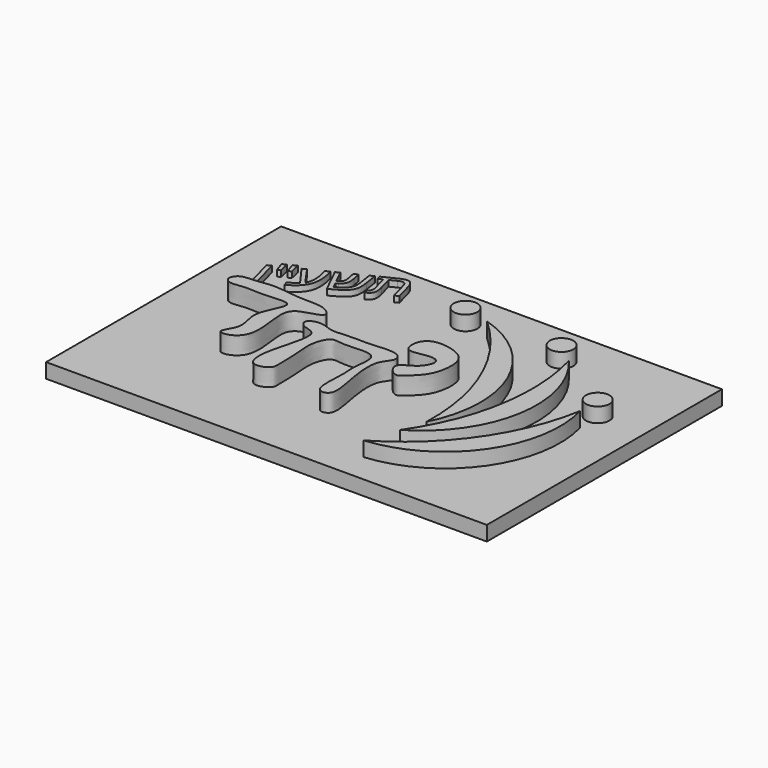
from build123d import *

# Parameters (mm, degrees)
F0_W         = 75
F0_H         = 50
F1_DEPTH     = 2.5
F2_R         = 2
F3_DEPTH     = 2.5
F5_DEPTH     = 3
F6_TEXT_SIZE = 8.2016766118
F7_DEPTH     = 1
F9_W         = 11.5771840792
F9_H         = 10.4032866075
F10_DEPTH    = 0.5


# Not quite as in the source:
# - Text() gives the source's letters only with a copy of the font that has no kerning and outlines rounded to 1/6400 em; it was checked with that copy


with BuildPart() as f1:
    # F0 (on Top) → F1 (new body)
    with BuildSketch(Plane.XY):
        Rectangle(F0_W, F0_H)
    extrude(amount=F1_DEPTH)

    # F2 (on face) → F3 (join)
    with BuildSketch(Plane.XY.offset(2.5)):
        with BuildLine():
            ThreePointArc((29.7072930905, 4.5745613287), (23.8276710869, -9.620101854), (12.5, -20))
            ThreePointArc((12.5, -20), (26.8332996169, -11.7246656078), (29.7072930905, 4.5745613287))
        make_face()
        with BuildLine():
            ThreePointArc((19.5, 14.9611591388), (20.2390516093, -0.3852482744), (14.4231878129, -14.6061535226))
            ThreePointArc((14.4231878129, -14.6061535226), (23.855326069, -1.0061753928), (19.5, 14.9611591388))
        make_face()
        with BuildLine():
            ThreePointArc((3.9204793744, 17), (12.8657059665, 4.5083492287), (15.6936347485, -10.5933472514))
            ThreePointArc((15.6936347485, -10.5933472514), (16.2405516301, 5.9482826301), (3.9204793744, 17))
        make_face()
        with Locations((29.4776950032, 8.6062820628)):
            Circle(F2_R)
        with Locations((15.9142967314, 17.8679712117)):
            Circle(F2_R)
        with Locations((-0.7517675404, 18.2841885835)):
            Circle(F2_R)
    extrude(amount=F3_DEPTH)

    # F4 (on face) → F5 (join)
    with BuildSketch(Plane.XY.offset(2.5)):
        with BuildLine():
            add(Edge.make_bspline(
                [(3.0326086562, -1.3369563967), (2.9350119626, -2.0403621451), (4.5917425614, -3.9939270927), (6.1221765899, -2.3629044841), (8.5639301497, -0.2651330915), (9.1837782901, 4.6769157571), (7.1382724113, 7.1335732235), (0.9439931643, 8.0903867753), (0.6074509574, 2.4736840768), (4.3394964182, 3.7996694306), (7.1189866446, 3.4381517938), (5.7369825883, 0.0853711506), (3.1405351803, -0.5591007677), (3.0326086562, -1.3369563967)],
                knots=[0, 0, 0, 0, 0.0820283677, 0.149981563, 0.2443794271, 0.3552738175, 0.4458566049, 0.5629281656, 0.6566670853, 0.7481320898, 0.8236216622, 0.9092895847, 1, 1, 1, 1], degree=3))
        make_face()
        with BuildLine():
            add(Edge.make_bspline(
                [(-8.1195654348, 1.4021738898), (-7.3091460708, 1.4638883512), (-5.5152173406, 1.4979414066), (-3.8993839761, 1.3561788354), (1.3062373781, 2.0276326248), (2.1890052278, -0.1990991053), (-0.1899071058, -2.0595975618), (0.8532602215, -8.5204361425), (1.8596445736, -13.170550048), (-1.4854668947, -13.5499339694), (-0.7054602406, -7.6018860046), (-1.2879564712, -5.0888774086), (-0.0704000749, 0.0848674398), (-6.1872854402, -1.1306872329), (-8.5713107205, -0.1164293629), (-9.8810248462, -3.3888872547), (-9.4053316768, -6.4864183569), (-9.3699151841, -10.7289633003), (-9.3291053367, -11.7402830835), (-10.5490449096, -12.7272870283), (-12.7365451038, -12.8700049727), (-13.4214275677, -8.8689190602), (-10.0259026165, -0.3658995166), (-13.6065604524, -0.3404836982), (-14.8001649364, 1.2876260355), (-12.4736171023, 2.432965484), (-10.1514072478, 1.1525955631), (-8.8514181621, 1.3464423774), (-8.1195654348, 1.4021738898)],
                knots=[0, 0, 0, 0, 0.0356309084, 0.066752293, 0.1164750348, 0.1443496844, 0.1795745535, 0.2376893049, 0.2839248957, 0.3122488532, 0.3627081661, 0.4035766295, 0.4464921147, 0.4962872854, 0.5304768764, 0.5675470115, 0.6100181617, 0.6558998739, 0.6776327498, 0.7043675142, 0.7332745461, 0.7760339489, 0.8400338198, 0.8742405934, 0.9006958848, 0.931635701, 0.9678233534, 1, 1, 1, 1], degree=3))
        make_face()
        with BuildLine():
            add(Edge.make_bspline(
                [(-23.7717386335, 6.4891306683), (-22.3277892961, 6.4818802962), (-19.212889904, 5.7552304549), (-14.9389873788, 6.2719279972), (-12.3476791544, 3.6958577814), (-18.258333606, 3.2432532034), (-18.0644065248, -0.9476344538), (-17.0828278202, -6.7668196304), (-20.1532019706, -8.5490693808), (-22.0136110622, -8.1310990471), (-19.3569725281, -5.1396286693), (-21.9046842163, -1.3803439435), (-17.4930362898, 4.5672265406), (-23.3641931196, 3.4702996666), (-26.5060886342, 4.0627689359), (-29.1572130934, 3.3225274488), (-30.3845535534, 4.5413152421), (-29.3017678601, 6.2062237341), (-27.0409204087, 6.0342583904), (-25.0073261179, 6.495334812), (-23.7717386335, 6.4891306683)],
                knots=[0, 0, 0, 0, 0.068199932, 0.134659527, 0.177792955, 0.2408170416, 0.3008700712, 0.3761845604, 0.4303485788, 0.4624548362, 0.5154515643, 0.5806868321, 0.6502993961, 0.7113339026, 0.7722981718, 0.8221058932, 0.8571571918, 0.8956899352, 0.9416413165, 1, 1, 1, 1], degree=3))
        make_face()
    extrude(amount=F5_DEPTH)

    # F6 (on face) → F7 (join)
    with BuildSketch(Plane.XY.offset(2.5)):
        with Locations(Location((-29.8022135976, 8.6265812861), (0, 0, 26.2432002765))):
            Text('ו"עשת', F6_TEXT_SIZE, font='Arimo', font_style=FontStyle.ITALIC, text_align=(TextAlign.LEFT, TextAlign.BOTTOM))
    extrude(amount=F7_DEPTH)

    # F9 (on face) → F10 (cut)
    with BuildSketch(Plane(origin=(0, 0, 0), x_dir=(1, 0, 0), z_dir=(0, 0, -1))):
        with Locations((1.9054870354, 4.319574713)):
            Rectangle(F9_W, F9_H)
    extrude(amount=-F10_DEPTH, mode=Mode.SUBTRACT)


solid = f1.part
